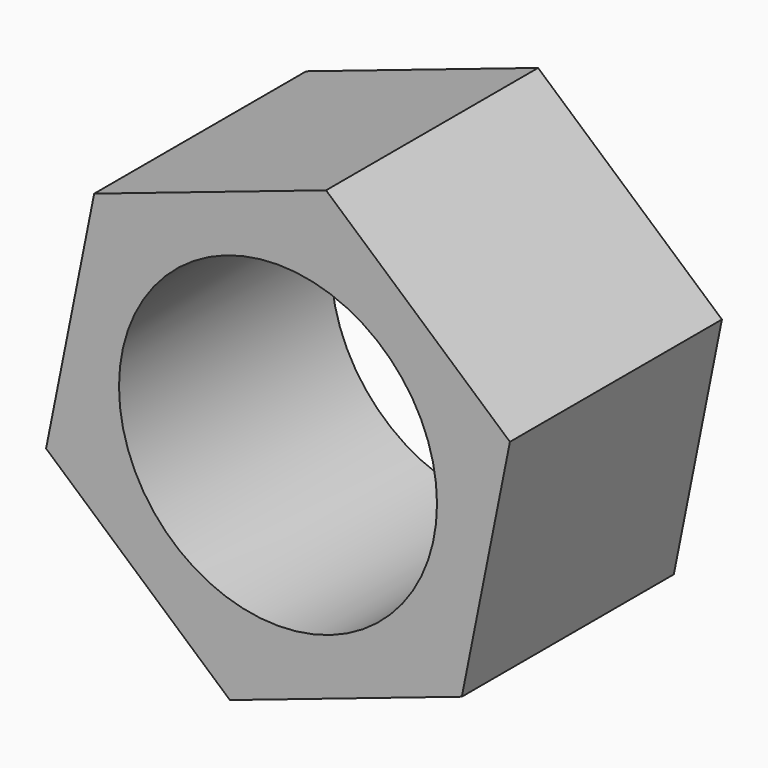
from build123d import *

# Parameters (mm, degrees)
F0_R     = 6
F1_DEPTH = 10


# Not quite as in the source:
# - the program builds the solid bodies; features that only make, move or delete a surface that nothing else refers to are left out


with BuildPart() as f1:
    # F0 (on Front) → F1 (new body)
    with BuildSketch(Plane.XZ):
        Polygon((-16.8017068945, -5.2552340917), (-8.0502918376, -2.2978589318), (-6.2357463262, 6.7597764064), (-13.1726158716, 12.8600365847), (-21.9240309284, 9.9026614248), (-23.7385764399, 0.8450260866), align=None)
        with Locations((-14.987161383, 3.8024012465)):
            Circle(F0_R, mode=Mode.SUBTRACT)
    extrude(amount=F1_DEPTH)


solid = f1.part
